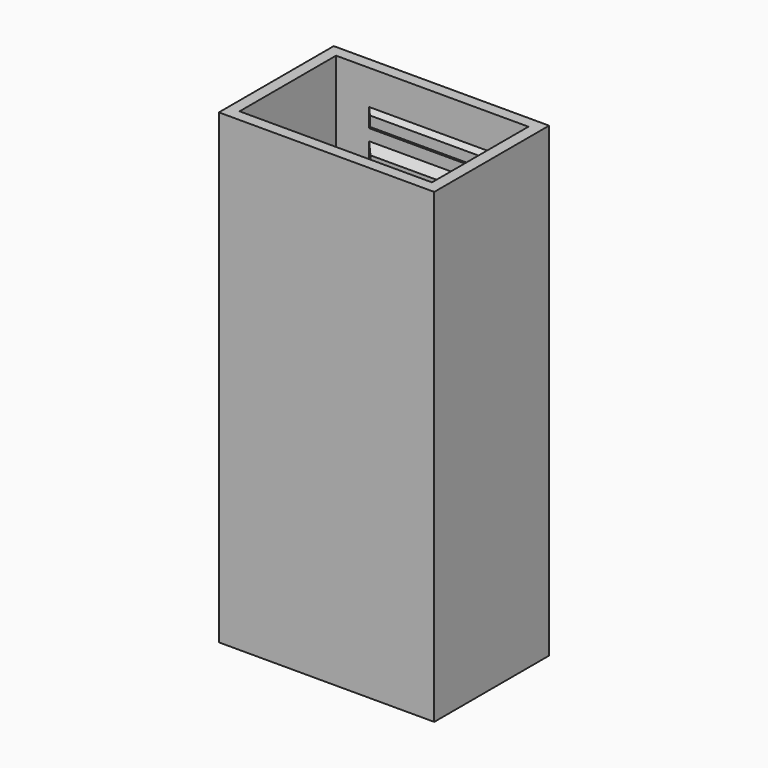
from build123d import *

# Parameters (mm, degrees)
F0_W         = 30
F0_H         = 20
F1_DEPTH     = 65
F0_W_2       = 23.6
F0_H_2       = 13.6
F0_W_3       = 16.8
F0_H_3       = 1
F2_DEPTH     = 1.5
F4_W         = 0.6
F4_H         = 3
F4_W_2       = 1
F4_H_2       = 4
F5_DEPTH     = 9
F6_T4_DEPTH  = 22.1146927807
F6_T9_DEPTH  = 22.1146927807
F6_T14_DEPTH = 7.1146927807
F6_T19_DEPTH = 7.1146927807
F7_T4_DEPTH  = 24.1720391711
F7_T9_DEPTH  = 24.1720391711
F7_T14_DEPTH = 10.1720391711
F7_T19_DEPTH = 10.1720391711


# Not quite as in the source:
# - a fillet or chamfer that OpenCascade refuses, or shapes differently, is made with other operations: its cross-section is extruded or revolved along the edge and cut away or added


with BuildPart() as f1:
    # F0 (on Top) → F1 (new body)
    with BuildSketch(Plane.XY):
        with Locations((-75, 70)):
            Rectangle(F0_W, F0_H)
        Polygon((-88.4, 61.6), (-88.4, 78.4), (-83.4, 78.4), (-66.6, 78.4), (-61.6, 78.4), (-61.6, 61.6), align=None, mode=Mode.SUBTRACT)
    extrude(amount=F1_DEPTH)

    # F0 (on Top) → F2 (join)
    with BuildSketch(Plane.XY):
        Polygon((-83.4, 78.4), (-88.4, 78.4), (-88.4, 61.6), (-61.6, 61.6), (-61.6, 78.4), (-66.6, 78.4), (-66.6, 77.4), (-83.4, 77.4), align=None)
        with Locations((-75, 70)):
            Rectangle(F0_W_2, F0_H_2, mode=Mode.SUBTRACT)
        with Locations((-75, 77.9)):
            Rectangle(F0_W_3, F0_H_3)
    extrude(amount=F2_DEPTH)

    # F4 (on mid) → F5 (join, symmetric)
    with BuildSketch(Plane.YZ.offset(-75)):
        with Locations((78.1, 58.9)):
            Rectangle(F4_W, F4_H)
        with Locations((77.9, 54.2)):
            Rectangle(F4_W_2, F4_H_2)
    extrude(amount=F5_DEPTH, both=True)

    # F6: chamfer of 0.8 on 4 edges, made by hand


with BuildPart() as f6_tool2:
    # F6_s3 → F6_t4 (new body)
    with BuildSketch(Plane.YZ.offset(-86.0573463904)):
        Polygon((78.6, 60.4), (77.8, 59.6), (77.8, 60.4), align=None)
    extrude(amount=F6_T4_DEPTH)

    split(bisect_by=Plane.XZ.offset(-78.4), keep=Keep.TOP)


with BuildPart() as f1_1:
    add(f1.part)

    # F6_t1: cut F6_tool2
    add(f6_tool2.part, mode=Mode.SUBTRACT)


with BuildPart() as f6_tool7:
    # F6_s8 → F6_t9 (new body)
    with BuildSketch(Plane.YZ.offset(-63.9426536096)):
        Polygon((78.6, 57.4), (77.8, 58.2), (77.8, 57.4), align=None)
    extrude(amount=-F6_T9_DEPTH)

    split(bisect_by=Plane.XZ.offset(-78.4), keep=Keep.TOP)


with BuildPart() as f1_2:
    add(f1_1.part)

    # F6_t6: cut F6_tool7
    add(f6_tool7.part, mode=Mode.SUBTRACT)


with BuildPart() as f6_tool12:
    # F6_s13 → F6_t14 (new body)
    with BuildSketch(Plane.XY.offset(62.4573463904)):
        Polygon((-84, 78.6), (-83.2, 77.8), (-84, 77.8), align=None)
    extrude(amount=-F6_T14_DEPTH)

    split(bisect_by=Plane.XZ.offset(-78.4), keep=Keep.TOP)


with BuildPart() as f1_3:
    add(f1_2.part)

    # F6_t11: cut F6_tool12
    add(f6_tool12.part, mode=Mode.SUBTRACT)


with BuildPart() as f6_tool17:
    # F6_s18 → F6_t19 (new body)
    with BuildSketch(Plane.XY.offset(62.4573463904)):
        Polygon((-66, 78.6), (-66.8, 77.8), (-66, 77.8), align=None)
    extrude(amount=-F6_T19_DEPTH)

    split(bisect_by=Plane.XZ.offset(-78.4), keep=Keep.TOP)


with BuildPart() as f1_4:
    add(f1_3.part)

    # F6_t16: cut F6_tool17
    add(f6_tool17.part, mode=Mode.SUBTRACT)

    # F7: chamfer of 1.2 on 4 edges, made by hand


with BuildPart() as f7_tool2:
    # F7_s3 → F7_t4 (new body)
    with BuildSketch(Plane.YZ.offset(-87.0860195856)):
        Polygon((78.6, 56.2), (77.4, 55), (77.4, 56.2), align=None)
    extrude(amount=F7_T4_DEPTH)

    split(bisect_by=Plane.XZ.offset(-78.4), keep=Keep.TOP)


with BuildPart() as f1_5:
    add(f1_4.part)

    # F7_t1: cut F7_tool2
    add(f7_tool2.part, mode=Mode.SUBTRACT)


with BuildPart() as f7_tool7:
    # F7_s8 → F7_t9 (new body)
    with BuildSketch(Plane.YZ.offset(-62.9139804144)):
        Polygon((78.6, 52.2), (77.4, 53.4), (77.4, 52.2), align=None)
    extrude(amount=-F7_T9_DEPTH)

    split(bisect_by=Plane.XZ.offset(-78.4), keep=Keep.TOP)


with BuildPart() as f1_6:
    add(f1_5.part)

    # F7_t6: cut F7_tool7
    add(f7_tool7.part, mode=Mode.SUBTRACT)


with BuildPart() as f7_tool12:
    # F7_s13 → F7_t14 (new body)
    with BuildSketch(Plane.XY.offset(59.2860195856)):
        Polygon((-84, 78.6), (-82.8, 77.4), (-84, 77.4), align=None)
    extrude(amount=-F7_T14_DEPTH)

    split(bisect_by=Plane.XZ.offset(-78.4), keep=Keep.TOP)


with BuildPart() as f1_7:
    add(f1_6.part)

    # F7_t11: cut F7_tool12
    add(f7_tool12.part, mode=Mode.SUBTRACT)


with BuildPart() as f7_tool17:
    # F7_s18 → F7_t19 (new body)
    with BuildSketch(Plane.XY.offset(59.2860195856)):
        Polygon((-66, 78.6), (-67.2, 77.4), (-66, 77.4), align=None)
    extrude(amount=-F7_T19_DEPTH)

    split(bisect_by=Plane.XZ.offset(-78.4), keep=Keep.TOP)


with BuildPart() as f1_8:
    add(f1_7.part)

    # F7_t16: cut F7_tool17
    add(f7_tool17.part, mode=Mode.SUBTRACT)


solid = f1_8.part
